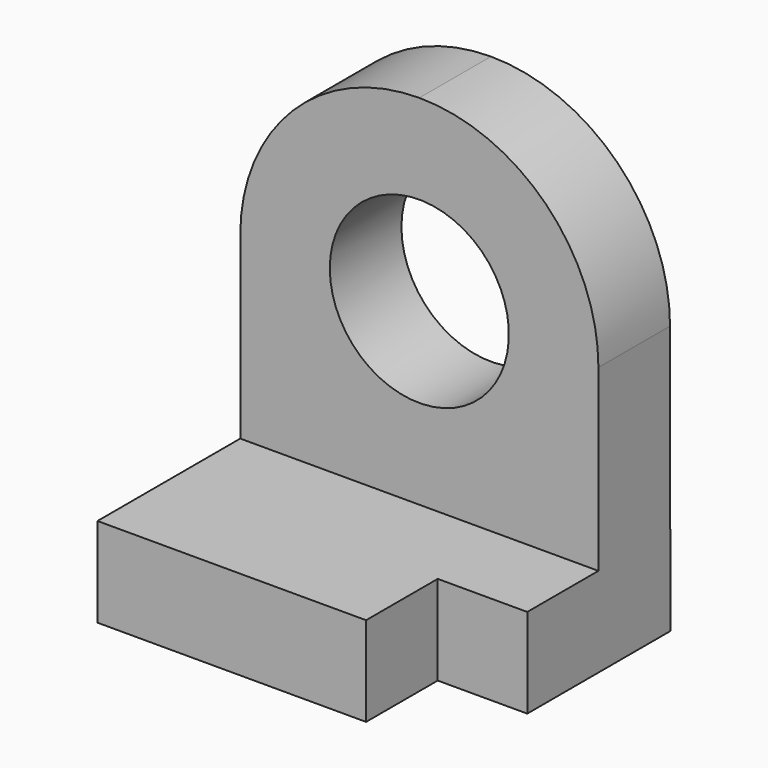
from build123d import *

# Parameters (mm, degrees)
F0_W     = 50.8
F0_H     = 38.1
F1_DEPTH = 12.7
F2_W     = 12.7
F2_H     = 12.7
F3_DEPTH = 12.7
F4_W     = 12.7
F4_H     = 50.8
F5_DEPTH = 50.8
F6_R     = 12.7
F7_DEPTH = 12.7
F8_R     = 25.4
F9_R     = 25.39999


# Not quite as in the source:
# - a fillet or chamfer is up to 0.001 mm smaller than in the source, because OpenCascade refuses the exact size


with BuildPart() as f1:
    # F0 (on Top) → F1 (new body)
    with BuildSketch(Plane.XY):
        Rectangle(F0_W, F0_H)
    extrude(amount=F1_DEPTH)

    # F2 (on face) → F3 (cut)
    with BuildSketch(Plane.XZ.offset(19.05)):
        with Locations((19.05, 6.35)):
            Rectangle(F2_W, F2_H)
    extrude(amount=-F3_DEPTH, mode=Mode.SUBTRACT)

    # F4 (on face) → F5 (join)
    with BuildSketch(Plane(origin=(-25.4, 0, 0), x_dir=(0, -1, 0), z_dir=(-1, 0, 0))):
        with Locations((-12.6142477781, 38.1)):
            Rectangle(F4_W, F4_H)
    extrude(amount=-F5_DEPTH)

    # F6 (on face) → F7 (cut)
    with BuildSketch(Plane(origin=(0, 18.9642477781, 0), x_dir=(-1, 0, 0), z_dir=(0, 1, 0))):
        with Locations((0, 38.1)):
            Circle(F6_R)
    extrude(amount=-F7_DEPTH, mode=Mode.SUBTRACT)

    # F8
    f8_edges = [f1.edges().sort_by_distance(p)[0] for p in [
        (-25.4, 12.614248, 63.5),
    ]]
    fillet(f8_edges, radius=F8_R)

    # F9 (radius 25.4 in the source; OpenCascade refuses exactly that, so slightly less here)
    f9_edges = [f1.edges().sort_by_distance(p)[0] for p in [
        (25.4, 12.614248, 63.5),
    ]]
    fillet(f9_edges, radius=F9_R)


solid = f1.part
